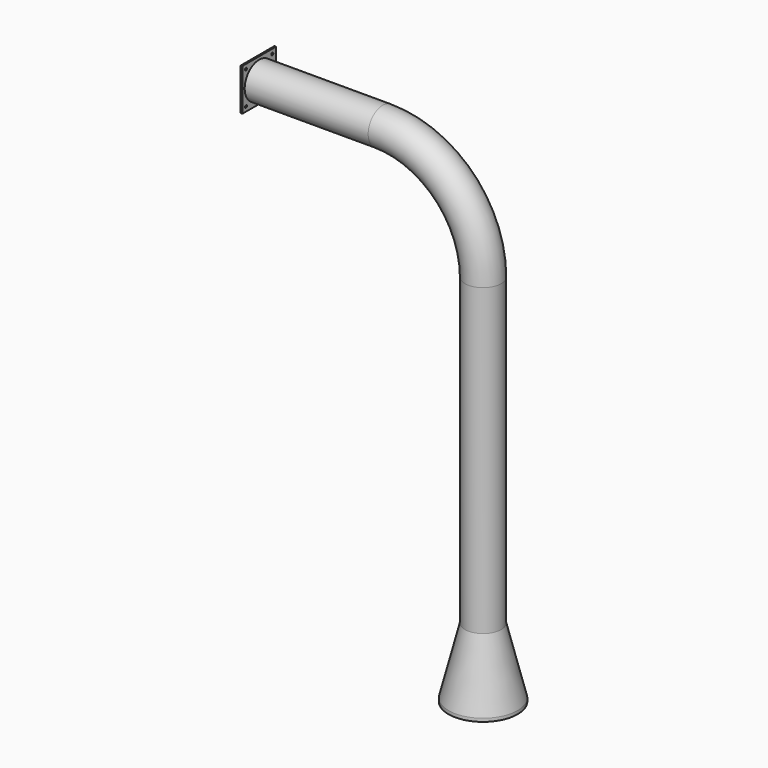
from build123d import *

# Parameters (mm, degrees)
F0_W       = 255
F0_H       = 255
F1_DEPTH   = 10
F2_D       = 15
F3_R       = 110
F4_DEPTH   = 750
F5_R       = 110
F6_ANGLE   = 90
F7_DEPTH   = 1850
F9_R       = 210
F10_DEPTH  = 20
F10_FACE_R = 210
F7_FACE_R  = 110


with BuildPart() as f1:
    # F0 (on Right) → F1 (new body)
    with BuildSketch(Plane.YZ):
        with Locations((67.6799364388, 95.7790961489)):
            Rectangle(F0_W, F0_H)
    extrude(amount=F1_DEPTH)

    # F2 (through all)
    with Locations(Plane(origin=(0, 0, 0), x_dir=(0, 1, 0), z_dir=(-1, 0, 0))):
        with Locations((-32.3200635612, -195.7790961489), (167.6799364388, -195.7790961489), (167.6799364388, 4.2209038511), (-32.3200635612, 4.2209038511)):
            Hole(F2_D / 2)

    # F3 (on face) → F4 (join)
    with BuildSketch(Plane.YZ.offset(10)):
        with Locations((67.6799364388, 95.7790961489)):
            Circle(F3_R)
    extrude(amount=F4_DEPTH)

    # F5 (on face) → F6 (revolve)
    with BuildSketch(Plane.YZ.offset(760)):
        with Locations((67.6799364388, 95.7790961489)):
            Circle(F5_R)
    revolve(axis=Axis((760, 94.2381992936, -514.2209038511), (0, 1, 0)), revolution_arc=F6_ANGLE)

    # F7 (add): a face of the model
    f7_faces = [f1.faces().sort_by_distance(p)[0] for p in [
        (1370, 67.6799364388, -514.2209038511),
    ]]
    extrude(f7_faces, amount=F7_DEPTH)


with BuildPart() as f10:
    # F9 (on face) → F10 (new body)
    with BuildSketch(Plane(origin=(0, 0, -2764.2209038511), x_dir=(1, 0, 0), z_dir=(0, 0, -1))):
        with Locations((1370, -67.6799364388)):
            Circle(F9_R)
    extrude(amount=F10_DEPTH)


with BuildPart() as f11:
    # F10_face (on face) → F11 section 0
    with BuildSketch(Plane(origin=(1370, 67.6799364388, -2764.2209038511), x_dir=(1, 0, 0), z_dir=(0, 0, 1))):
        Circle(F10_FACE_R)
    # F7_face (on face) → F11 section 1
    with BuildSketch(Plane(origin=(1370, 67.6799364388, -2364.2209038511), x_dir=(1, 0, 0), z_dir=(0, 0, -1))):
        Circle(F7_FACE_R)
    loft()


solid = Compound([f1.part, f10.part, f11.part])
